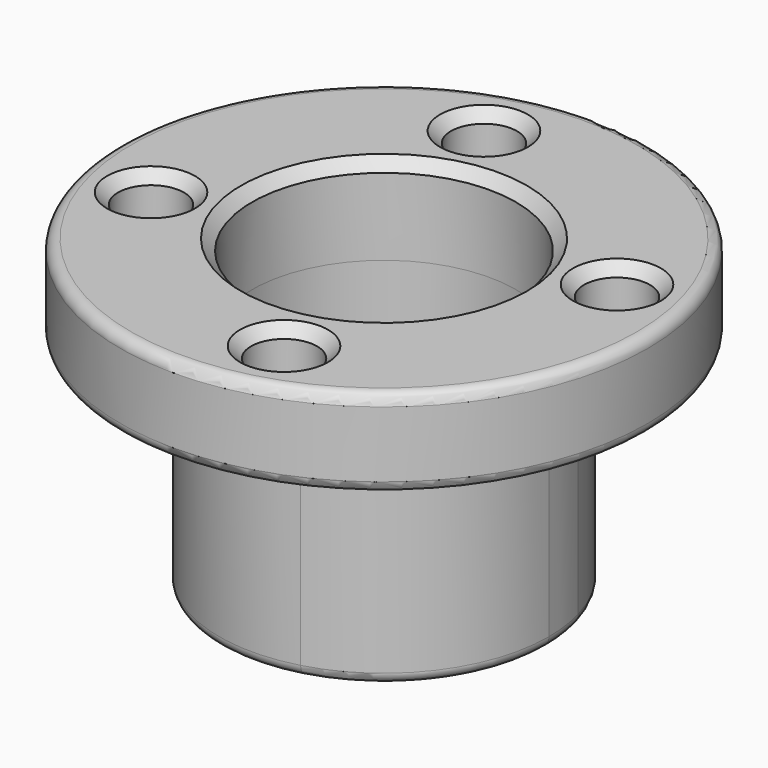
from build123d import *

# Parameters (mm, degrees)
F0_R           = 6
F0_R_2         = 3
F1_DEPTH       = 2
F2_D           = 1.5
F2_CSINK_D     = 2
F2_CSINK_ANGLE = 90
F3_SIZE        = 0.25
F4_R           = 3
F5_DEPTH       = 5
F6_R           = 0.25
F7_R           = 0.25


with BuildPart() as f1:
    # F0 (on Top) → F1 (new body)
    with BuildSketch(Plane.XY):
        Circle(F0_R)
        Circle(F0_R_2, mode=Mode.SUBTRACT)
    extrude(amount=-F1_DEPTH)

    # F2 (through all)
    with Locations(Plane.XY):
        with Locations((-1.1978440184, 4.3376456411), (1.1978440184, -4.3376456411), (-4.3376456411, -1.1978440184), (4.3376456411, 1.1978440184)):
            CounterSinkHole(F2_D / 2, F2_CSINK_D / 2, counter_sink_angle=F2_CSINK_ANGLE)

    # F3
    f3_edges = [f1.edges().sort_by_distance(p)[0] for p in [
        (-3, 0, 0),
    ]]
    chamfer(f3_edges, length=F3_SIZE)

    # F4 (on face) → F5 (join)
    with BuildSketch(Plane(origin=(0, 0, -2), x_dir=(1, 0, 0), z_dir=(0, 0, -1))):
        with BuildLine():
            ThreePointArc((3.6147047033, -0.99820334), (3.7160222441, -0.5036652473), (3.75, 0))
            ThreePointArc((3.75, 0), (2.9837696475, 2.2714794057), (0.9982033651, 3.6147046964))
            ThreePointArc((0.9982033651, 3.6147046964), (-1.8501458456, 3.2618185648), (-3.6147047033, 0.99820334))
            ThreePointArc((-3.6147047033, 0.99820334), (-3.2618185584, -1.850145857), (-0.99820334, -3.6147047033))
            ThreePointArc((-0.99820334, -3.6147047033), (1.850145857, -3.2618185584), (3.6147047033, -0.99820334))
        make_face()
        Circle(F4_R, mode=Mode.SUBTRACT)
    extrude(amount=F5_DEPTH)

    # F6
    f6_edges = [f1.edges().sort_by_distance(p)[0] for p in [
        (-3, 0, -7),
        (-3.614705, -0.998203, -7),
    ]]
    fillet(f6_edges, radius=F6_R)

    # F7
    f7_edges = [f1.edges().sort_by_distance(p)[0] for p in [
        (-6, 0, 0),
        (-6, 0, -2),
    ]]
    fillet(f7_edges, radius=F7_R)


solid = f1.part
